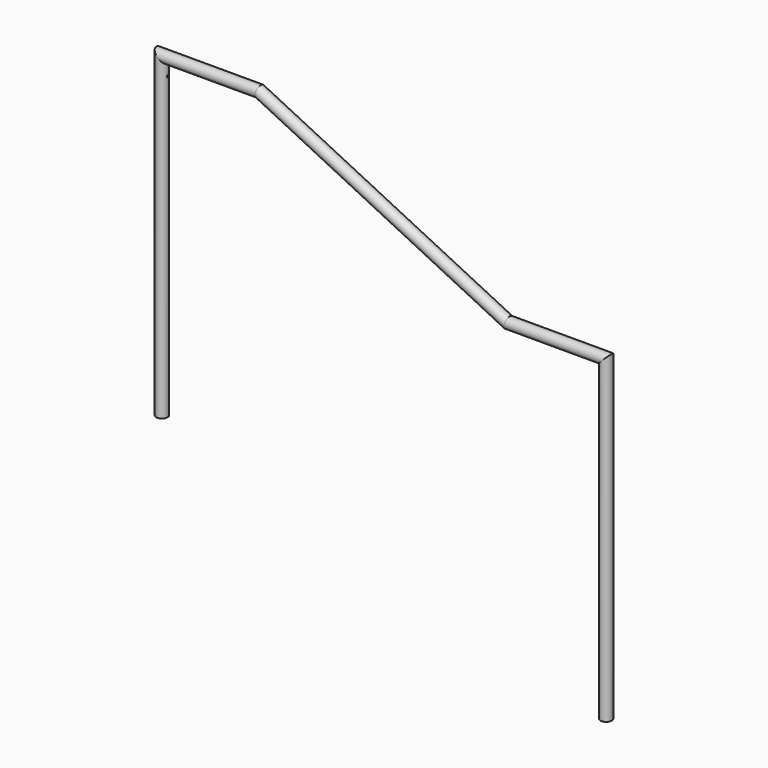
from build123d import *

# Parameters (mm, degrees)
F2_R      = 19.05
F9_D      = 6.35
F9_DEPTH  = 12.7
F9_TIP    = 1.9077324654
F15_D     = 6.35
F15_DEPTH = 12.7
F15_TIP   = 1.9077324654


with BuildPart() as f3:
    # F3: sweep along a path in F0
    with BuildLine(Plane.XZ) as f3_path:
        Line((-626.3162476942, -437.036204844), (-626.3162476942, 629.763795156))
        Line((-626.3162476942, 629.763795156), (-298.0212476942, 629.763795156))
        Line((-298.0212476942, 629.763795156), (539.3806681667, 217.3478233358))
        Line((539.3806681667, 217.3478233358), (867.6756681667, 217.3478233358))
        Line((867.6756681667, 217.3478233358), (867.6756681667, -849.4521766642))
    # F2 (on plane+point) → F3 (sweep)
    with BuildSketch(Plane.XY.offset(-437.036204844)):
        with Locations((-626.3162476942, 0)):
            Circle(F2_R)
    sweep(path=f3_path.line, transition=Transition.RIGHT)

    # F9 (one way)
    with BuildSketch(Plane.YZ.offset(-607.2662476942)):
        with Locations((0, 572.613795156)):
            Circle(F9_D / 2)
    extrude(amount=-F9_DEPTH, mode=Mode.SUBTRACT)
    with Locations(Plane.YZ.offset(-607.2662476942)):
        with Locations((0, 572.613795156)):
            with Locations((0, 0, -(F9_DEPTH + F9_TIP / 2))):  # 118° drill point
                Cone(0, F9_D / 2, F9_TIP, mode=Mode.SUBTRACT)

    # F15 (one way)
    with BuildSketch(Plane(origin=(848.6256681667, 0, 0), x_dir=(0, -1, 0), z_dir=(-1, 0, 0))):
        with Locations((0, 160.1978233358)):
            Circle(F15_D / 2)
    extrude(amount=-F15_DEPTH, mode=Mode.SUBTRACT)
    with Locations(Plane(origin=(848.6256681667, 0, 0), x_dir=(0, -1, 0), z_dir=(-1, 0, 0))):
        with Locations((0, 160.1978233358)):
            with Locations((0, 0, -(F15_DEPTH + F15_TIP / 2))):  # 118° drill point
                Cone(0, F15_D / 2, F15_TIP, mode=Mode.SUBTRACT)


solid = f3.part
